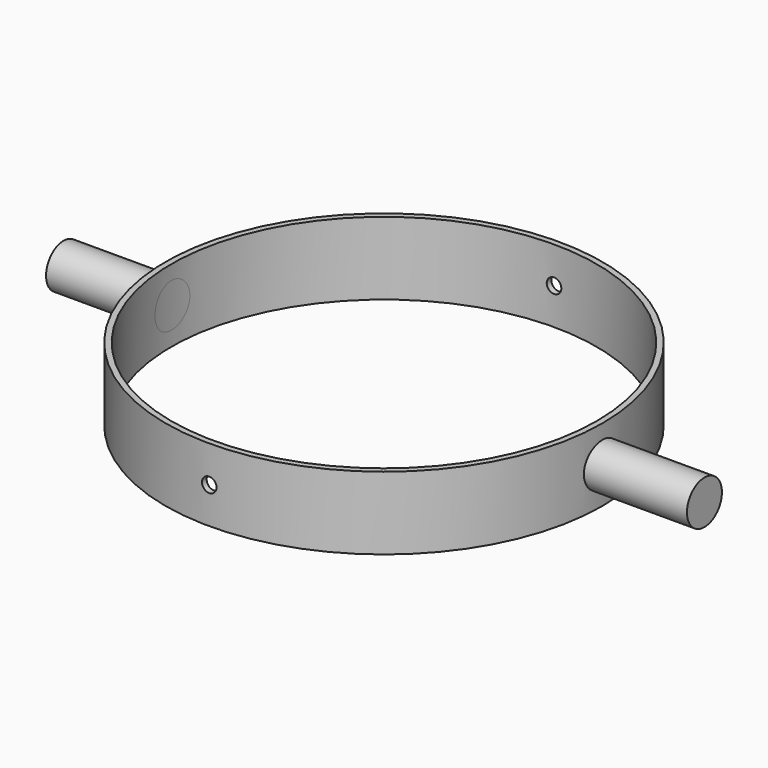
from build123d import *

# Parameters (mm, degrees)
F0_R     = 75
F0_R_2   = 73
F1_DEPTH = 12.5
F2_R     = 2.5
F3_DEPTH = 75.001
F4_DEPTH = 75.0010001
F5_R     = 7.5
F6_DEPTH = 110
F7_REACH = 131.2142034356


with BuildPart() as f1:
    # F0 (on Top) → F1 (new body, symmetric)
    with BuildSketch(Plane.XY):
        Circle(F0_R)
        Circle(F0_R_2, mode=Mode.SUBTRACT)
    extrude(amount=F1_DEPTH, both=True)

    # F2 (on Front) → F3 (cut, through all)
    with BuildSketch(Plane.XZ):
        Circle(F2_R)
    extrude(amount=-F3_DEPTH, mode=Mode.SUBTRACT)

    # F2 (on Front) → F4 (cut, through all)
    with BuildSketch(Plane.XZ):
        Circle(F2_R)
    extrude(amount=F4_DEPTH, mode=Mode.SUBTRACT)


with BuildPart() as f6:
    # F5 (on Right) → F6 (new body)
    with BuildSketch(Plane.YZ):
        Circle(F5_R)
    extrude(amount=F6_DEPTH)

    f7_end = f1.part.faces().sort_by_distance((-73, 0, 0))[0]
    # F5 (on Right) → F7 (cut, up to a face of F1 that its end follows)
    with BuildSketch(Plane.YZ):
        Circle(F5_R)
    f7_long = extrude(amount=F7_REACH, mode=Mode.PRIVATE)
    add(split(f7_long, bisect_by=f7_end, keep=Keep.TOP, mode=Mode.PRIVATE), mode=Mode.SUBTRACT)


with BuildPart() as f1_1:
    add(f1.part)

    add(f6.part)  # F8 merges F6
    # F8: F6 across plane
    add(f6.part.mirror(Plane.YZ))


solid = f1_1.part
